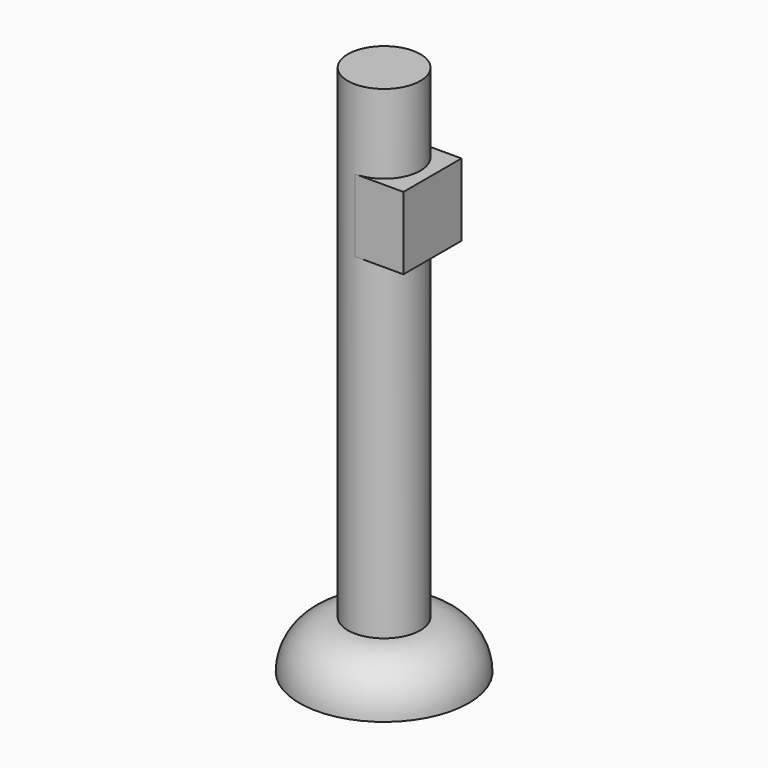
from build123d import *

# Parameters (mm, degrees)
F0_R     = 44.45
F1_DEPTH = 25.4
F2_R     = 25.39999
F3_DEPTH = 254
F4_W     = 38.1
F4_H     = 38.1
F5_DEPTH = 25.4


# Not quite as in the source:
# - a fillet or chamfer is up to 0.001 mm smaller than in the source, because OpenCascade refuses the exact size


with BuildPart() as f1:
    # F0 (on Top) → F1 (new body)
    with BuildSketch(Plane.XY):
        Circle(F0_R)
    extrude(amount=F1_DEPTH)

    # F2 (radius 25.4 in the source; OpenCascade refuses exactly that, so slightly less here)
    f2_edges = [f1.edges().sort_by_distance(p)[0] for p in [
        (-44.45, 0, 25.4),
    ]]
    fillet(f2_edges, radius=F2_R)

    # F3 (add): a face of the model
    f3_faces = [f1.faces().sort_by_distance(p)[0] for p in [
        (0, 0, 25.4),
    ]]
    extrude(f3_faces, amount=F3_DEPTH)

    # F4 (on Right) → F5 (join)
    with BuildSketch(Plane.YZ):
        with Locations((0, 218.8449014022)):
            Rectangle(F4_W, F4_H)
    extrude(amount=F5_DEPTH)


solid = f1.part
